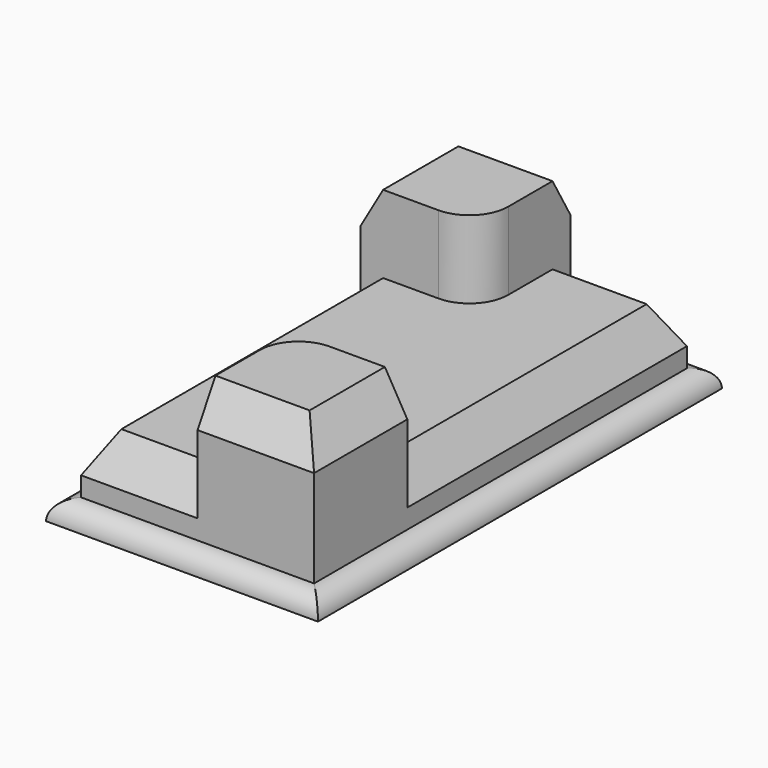
from build123d import *

# Parameters (mm, degrees)
F0_W     = 88.9
F0_H     = 165.1
F1_DEPTH = 6.35
F2_DEPTH = 25.4
F3_DEPTH = 50.8
F4_SIZE2 = 7.3323484187
F4_SIZE  = 12.7
F5_R     = 6.34999
F6_SIZE2 = 7.3323484187
F6_SIZE  = 12.7


# Not quite as in the source:
# - a fillet or chamfer is up to 0.001 mm smaller than in the source, because OpenCascade refuses the exact size


with BuildPart() as f1:
    # F0 (on Top) → F1 (new body)
    with BuildSketch(Plane.XY):
        Rectangle(F0_W, F0_H)
        Polygon((38.1, -38.1), (38.1, -76.2), (0, -76.2), (-38.1, -76.2), (-38.1, 38.1), (-38.1, 76.2), (0, 76.2), (38.1, 76.2), align=None, mode=Mode.SUBTRACT)
    extrude(amount=F1_DEPTH)

    # F0 (on Top) → F2 (join)
    with BuildSketch(Plane.XY):
        with BuildLine():
            Line((-38.1, -76.2), (0, -76.2))
            Line((0, -76.2), (0, -50.8))
            ThreePointArc((0, -50.8), (3.7197438789, -41.8197438789), (12.7, -38.1))
            Line((12.7, -38.1), (38.1, -38.1))
            Line((38.1, -38.1), (38.1, 76.2))
            Line((38.1, 76.2), (0, 76.2))
            Line((0, 76.2), (0, 50.8))
            ThreePointArc((0, 50.8), (-3.7197438789, 41.8197438789), (-12.7, 38.1))
            Line((-12.7, 38.1), (-38.1, 38.1))
            Line((-38.1, 38.1), (-38.1, -76.2))
        make_face()
    extrude(amount=F2_DEPTH)

    # F0 (on Top) → F3 (join)
    with BuildSketch(Plane.XY):
        with BuildLine():
            Line((-38.1, 76.2), (-38.1, 38.1))
            Line((-38.1, 38.1), (-12.7, 38.1))
            ThreePointArc((-12.7, 38.1), (-3.7197438789, 41.8197438789), (0, 50.8))
            Line((0, 50.8), (0, 76.2))
            Line((0, 76.2), (-38.1, 76.2))
        make_face()
        with BuildLine():
            Line((0, -76.2), (38.1, -76.2))
            Line((38.1, -76.2), (38.1, -38.1))
            Line((38.1, -38.1), (12.7, -38.1))
            ThreePointArc((12.7, -38.1), (3.7197438789, -41.8197438789), (0, -50.8))
            Line((0, -50.8), (0, -76.2))
        make_face()
    extrude(amount=F3_DEPTH)

    # F4
    f4_edges = [f1.edges().sort_by_distance(p)[0] for p in [
        (19.05, -76.2, 50.8),
        (38.1, -57.15, 50.8),
        (-19.05, -76.2, 25.4),
        (-38.1, -19.05, 25.4),
        (-38.1, 57.15, 50.8),
    ]]
    chamfer(f4_edges, length=F4_SIZE, length2=F4_SIZE2)

    # F5 (radius 6.35 in the source; OpenCascade refuses exactly that, so slightly less here)
    f5_edges = [f1.edges().sort_by_distance(p)[0] for p in [
        (0, 82.55, 6.35),
        (44.45, 0, 6.35),
        (-44.45, 0, 6.35),
        (0, -82.55, 6.35),
    ]]
    fillet(f5_edges, radius=F5_R)

    # F6
    f6_edges = [f1.edges().sort_by_distance(p)[0] for p in [
        (-12.7, 76.2, 50.8),
        (19.05, 76.2, 25.4),
        (38.1, 19.05, 25.4),
    ]]
    chamfer(f6_edges, length=F6_SIZE, length2=F6_SIZE2)


solid = f1.part
